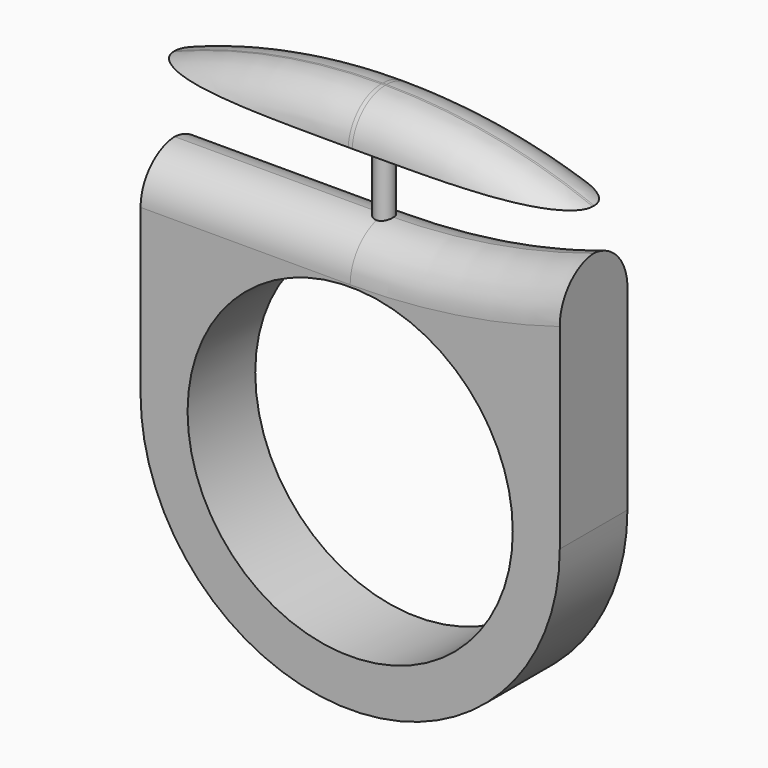
from build123d import *

# Parameters (mm, degrees)
F0_R          = 8.65
F1_DEPTH      = 2.25
F1_DEPTH_BACK = 2.25
F5_T1_DEPTH   = 59.7206593681
F6_T1_DEPTH   = 0.2117362528
F6_T4_ANGLE   = 31.7141074843
F6_T6_ANGLE   = 31.7141074843
F6_T8_ANGLE   = 31.7141074843
F6_T10_ANGLE  = 31.7141074843
F7_T3_DEPTH   = 17.15
F7_T6_DEPTH   = 17.15
F7_T9_ANGLE   = 27.8482361684
F7_T12_ANGLE  = 27.8482361684
F8_R          = 0.5
F9_DEPTH      = 2.2
F9_DEPTH_BACK = 2.2


# Not quite as in the source:
# - a fillet or chamfer that OpenCascade refuses, or shapes differently, is made with other operations: its cross-section is extruded or revolved along the edge and cut away or added
# - the program builds the solid bodies; features that only make, move or delete a surface that nothing else refers to are left out


with BuildPart() as f1:
    # F0 (on Front) → F1 (new body, two sides)
    with BuildSketch(Plane.XZ) as f1_sk:
        with BuildLine():
            ThreePointArc((-11.15, 0), (0, -11.15), (11.15, 0))
            ThreePointArc((11.15, 0), (7.8842406102, 7.8842406102), (0, 11.15))
            ThreePointArc((0, 11.15), (-7.8842406102, 7.8842406102), (-11.15, 0))
        make_face()
        Circle(F0_R, mode=Mode.SUBTRACT)
        with BuildLine():
            ThreePointArc((-11.15, 0), (-7.8842406102, 7.8842406102), (0, 11.15))
            Line((0, 11.15), (-4, 11.15))
            Line((-4, 11.15), (-9.15, 11.15))
            Line((-9.15, 11.15), (-11.15, 11.15))
            Line((-11.15, 11.15), (-11.15, 0))
        make_face()
        with BuildLine():
            ThreePointArc((0, 11.15), (7.8842406102, 7.8842406102), (11.15, 0))
            Line((11.15, 0), (11.15, 11.15))
            Line((11.15, 11.15), (0, 11.15))
        make_face()
        with BuildLine():
            ThreePointArc((11.15, 12.9371443763), (5.6461576541, 11.5996193357), (0, 11.15))
            Line((0, 11.15), (11.15, 11.15))
            Line((11.15, 11.15), (11.15, 12.9371443763))
        make_face()
    extrude(amount=F1_DEPTH)
    extrude(f1_sk.sketch, amount=-F1_DEPTH_BACK)

    # F7: fillet of radius 2.4 on 2 edges, made by hand


with BuildPart() as f1b:
    # F0 (on Front) → F1, piece 2 (new body, two sides)
    with BuildSketch(Plane.XZ) as f1_2_sk:
        Polygon((-9.15, 15.15), (-4, 15.15), (0, 15.15), (11.15, 15.15), (11.15, 17.2301754355), (-11.15, 17.2301754355), (-11.15, 15.15), align=None)
    extrude(amount=F1_DEPTH)
    extrude(f1_2_sk.sketch, amount=-F1_DEPTH_BACK)

    # F5: fillet of radius 30.3580112828 on 2 edges, made by hand

    # F5_s2 → F5_t1 (cut)
    with BuildSketch(Plane.XZ.offset(-29.8603296841)):
        with BuildLine():
            ThreePointArc((-0.1058681264, 17.2301754355), (-5.725031291, 16.7055993283), (-11.15, 15.15))
            Line((-11.15, 15.15), (-11.3708826375, 15.7155567169))
            ThreePointArc((-11.3708826375, 15.7155567169), (-11.7571602257, 16.1900877178), (-11.7571602257, 17.2301754355))
            Line((-11.7571602257, 17.2301754355), (-11.15, 17.8373356612))
            Line((-11.15, 17.8373356612), (-0.1058681264, 17.8373356612))
            Line((-0.1058681264, 17.8373356612), (-0.1058681264, 17.2301754355))
        make_face()
        with BuildLine():
            ThreePointArc((0.1058681264, 17.2301754355), (5.725031291, 16.7055993283), (11.15, 15.15))
            Line((11.15, 15.15), (11.3708826375, 15.7155567169))
            ThreePointArc((11.3708826375, 15.7155567169), (11.7571602257, 16.1900877178), (11.7571602257, 17.2301754355))
            Line((11.7571602257, 17.2301754355), (11.15, 17.8373356612))
            Line((11.15, 17.8373356612), (0.1058681264, 17.8373356612))
            Line((0.1058681264, 17.8373356612), (0.1058681264, 17.2301754355))
        make_face()
    extrude(amount=F5_T1_DEPTH, mode=Mode.SUBTRACT)

    # F6: fillet of radius 2.2 on 2 edges, made by hand

    # F6_s2 → F6_t1 (cut)
    with BuildSketch(Plane.YZ.offset(-0.1058681264)):
        with BuildLine():
            ThreePointArc((2.25, 15.0301754355), (1.6056349186, 16.5858103542), (0.05, 17.2301754355))
            Line((0.05, 17.2301754355), (2.25, 17.2301754355))
            Line((2.25, 17.2301754355), (2.25, 15.0301754355))
        make_face()
        with BuildLine():
            ThreePointArc((-2.25, 15.0301754355), (-1.6056349186, 16.5858103542), (-0.05, 17.2301754355))
            Line((-0.05, 17.2301754355), (-2.25, 17.2301754355))
            Line((-2.25, 17.2301754355), (-2.25, 15.0301754355))
        make_face()
    extrude(amount=F6_T1_DEPTH, mode=Mode.SUBTRACT)

    # F6_s3 → F6_t4 (revolve, cut)
    with BuildSketch(Plane(origin=(-5.9472140901, 0, -3.6750974915), x_dir=(0, 1, 0), z_dir=(-0.8506817009, 0, -0.5256811236))):
        with BuildLine():
            ThreePointArc((-0.05, -19.2460544304), (-1.6056349186, -18.601689349), (-2.25, -17.0460544304))
            Line((-2.25, -17.0460544304), (-2.25, -19.2460544304))
            Line((-2.25, -19.2460544304), (-0.05, -19.2460544304))
        make_face()
    revolve(axis=Axis((-0.1058681264, -2.25, -13.1278358476), (0, 1, 0)), revolution_arc=F6_T4_ANGLE, mode=Mode.SUBTRACT)

    # F6_s5 → F6_t6 (revolve, cut)
    with BuildSketch(Plane.YZ.offset(0.1058681264)):
        with BuildLine():
            ThreePointArc((0.05, 17.2301754355), (1.6056349186, 16.5858103541), (2.25, 15.0301754355))
            Line((2.25, 15.0301754355), (2.25, 17.2301754355))
            Line((2.25, 17.2301754355), (0.05, 17.2301754355))
        make_face()
    revolve(axis=Axis((0.1058681264, 2.25, -13.1278358476), (0, 1, 0)), revolution_arc=F6_T6_ANGLE, mode=Mode.SUBTRACT)

    # F6_s7 → F6_t8 (revolve, cut)
    with BuildSketch(Plane(origin=(-5.9472140901, 0, -3.6750974915), x_dir=(0, 1, 0), z_dir=(-0.8506817009, 0, -0.5256811236))):
        with BuildLine():
            ThreePointArc((0.05, -19.2460544304), (1.6056349186, -18.601689349), (2.25, -17.0460544304))
            Line((2.25, -17.0460544304), (2.25, -19.2460544304))
            Line((2.25, -19.2460544304), (0.05, -19.2460544304))
        make_face()
    revolve(axis=Axis((-0.1058681264, 2.25, -13.1278358476), (0, 1, 0)), revolution_arc=F6_T8_ANGLE, mode=Mode.SUBTRACT)

    # F6_s9 → F6_t10 (revolve, cut)
    with BuildSketch(Plane.YZ.offset(0.1058681264)):
        with BuildLine():
            ThreePointArc((-2.25, 15.0301754355), (-1.6056349186, 16.5858103541), (-0.05, 17.2301754355))
            Line((-0.05, 17.2301754355), (-2.25, 17.2301754355))
            Line((-2.25, 17.2301754355), (-2.25, 15.0301754355))
        make_face()
    revolve(axis=Axis((0.1058681264, -2.25, -13.1278358476), (0, 1, 0)), revolution_arc=F6_T10_ANGLE, mode=Mode.SUBTRACT)


with BuildPart() as f7_tool1:
    # F7_s2 → F7_t3 (new body)
    with BuildSketch(Plane.YZ):
        with BuildLine():
            ThreePointArc((0.15, 11.15), (-1.5470562748, 10.4470562748), (-2.25, 8.75))
            Line((-2.25, 8.75), (-2.25, 11.15))
            Line((-2.25, 11.15), (0.15, 11.15))
        make_face()
    extrude(amount=-F7_T3_DEPTH)


with BuildPart() as f7_tool4:
    # F7_s5 → F7_t6 (new body)
    with BuildSketch(Plane.YZ):
        with BuildLine():
            ThreePointArc((2.25, 8.75), (1.5470562748, 10.4470562748), (-0.15, 11.15))
            Line((-0.15, 11.15), (2.25, 11.15))
            Line((2.25, 11.15), (2.25, 8.75))
        make_face()
    extrude(amount=-F7_T6_DEPTH)


with BuildPart() as f7_tool7:
    # F7_s8 → F7_t9 (revolve)
    with BuildSketch(Plane(origin=(19.3406338701, 0, 10.217977433), x_dir=(0, 1, 0), z_dir=(0.8841880202, 0, 0.467131186))):
        with BuildLine():
            ThreePointArc((2.25, 3.3269863074), (1.5470562748, 5.0240425823), (-0.15, 5.7269863074))
            Line((-0.15, 5.7269863074), (2.25, 5.7269863074))
            Line((2.25, 5.7269863074), (2.25, 3.3269863074))
        make_face()
    revolve(axis=Axis((0, 2.25, 46.8260166415), (0, 1, 0)), revolution_arc=F7_T9_ANGLE)


with BuildPart() as f7_tool10:
    # F7_s11 → F7_t12 (revolve)
    with BuildSketch(Plane(origin=(19.3406338701, 0, 10.217977433), x_dir=(0, 1, 0), z_dir=(0.8841880202, 0, 0.467131186))):
        with BuildLine():
            ThreePointArc((0.15, 5.7269863074), (-1.5470562748, 5.0240425823), (-2.25, 3.3269863074))
            Line((-2.25, 3.3269863074), (-2.25, 5.7269863074))
            Line((-2.25, 5.7269863074), (0.15, 5.7269863074))
        make_face()
    revolve(axis=Axis((0, -2.25, 46.8260166415), (0, 1, 0)), revolution_arc=F7_T12_ANGLE)


with BuildPart() as f1_1:
    add(f1.part)

    # F7_t13: cut F7_tool1, F7_tool4, F7_tool7, F7_tool10
    add([f7_tool1.part, f7_tool4.part, f7_tool7.part, f7_tool10.part], mode=Mode.SUBTRACT)


with BuildPart() as f9:
    # F8 (on offset) → F9 (new body, two sides)
    with BuildSketch(Plane.XY.offset(13.15)) as f9_sk:
        Circle(F8_R)
    extrude(amount=F9_DEPTH)
    extrude(f9_sk.sketch, amount=-F9_DEPTH_BACK)


solid = Compound([f1b.part, f1_1.part, f9.part])
